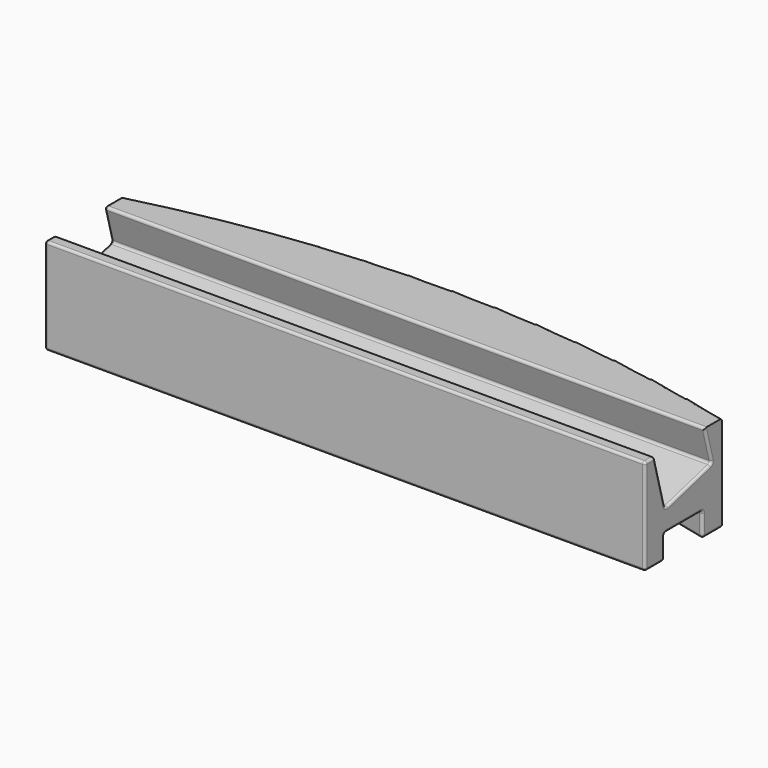
from build123d import *

# Parameters (mm, degrees)
F1_DEPTH = 40
F3_DEPTH = 250.001
F5_DEPTH = 10
F6_R     = 1


with BuildPart() as f1:
    # F0 (on Top) → F1 (new body)
    with BuildSketch(Plane.XY):
        with BuildLine():
            Line((-125, 40), (-125, 0))
            Line((-125, 0), (125, 0))
            Line((125, 0), (125, 40))
            ThreePointArc((125, 40), (0, 55.8770817241), (-125, 40))
        make_face()
    extrude(amount=F1_DEPTH)

    # F2 (on face) → F3 (cut, through all)
    with BuildSketch(Plane.YZ.offset(125)):
        Polygon((5, 40), (10.6160445296, 19.0406364781), (34.7641901868, 25.5111126057), (30.8819045103, 40), align=None)
    extrude(amount=-F3_DEPTH, mode=Mode.SUBTRACT)

    # F4 (on face) → F5 (cut)
    with BuildSketch(Plane(origin=(0, 0, 0), x_dir=(1, 0, 0), z_dir=(0, 0, -1))):
        with BuildLine():
            ThreePointArc((-125, -29.6650089658), (0, -45.8770817241), (125, -29.6650089658))
            Line((125, -29.6650089658), (125, -10))
            Line((125, -10), (-125, -10))
            Line((-125, -10), (-125, -29.6650089658))
        make_face()
    extrude(amount=-F5_DEPTH, mode=Mode.SUBTRACT)

    # F6
    f6_edges = [f1.edges().sort_by_distance(p)[0] for p in [
        (0, 55.877082, 40),
        (0, 30.881905, 40),
        (-125, 35.440952, 40),
        (-125, 34.832504, 0),
        (-125, 29.665009, 5),
        (-125, 19.832504, 10),
        (-125, 10, 5),
        (-125, 5, 0),
        (-125, 0, 20),
        (-125, 2.5, 40),
        (-125, 7.808022, 29.520318),
        (-125, 22.690117, 22.275875),
        (-125, 32.823047, 32.755556),
        (-125, 40, 20),
        (125, 22.690117, 22.275875),
        (0, 34.76419, 25.511113),
        (0, 10.616045, 19.040636),
        (125, 2.5, 40),
        (0, 0, 40),
        (0, 5, 40),
        (0, 45.877082, 10),
        (125, 19.832504, 10),
        (0, 10, 10),
        (125, 29.665009, 5),
        (0, 45.877082, 0),
        (125, 34.832504, 0),
        (0, 55.877082, 0),
        (125, 5, 0),
        (0, 0, 0),
        (0, 10, 0),
        (125, 0, 20),
        (125, 10, 5),
        (125, 32.823047, 32.755556),
        (125, 7.808022, 29.520318),
    ]]
    fillet(f6_edges, radius=F6_R)


solid = f1.part
